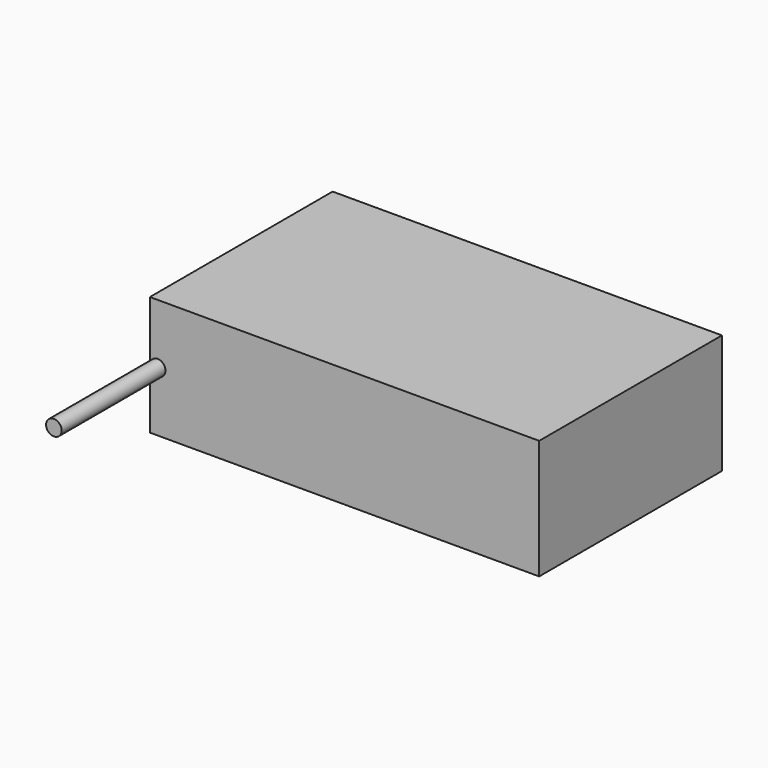
from build123d import *

# Parameters (mm, degrees)
F1_DEPTH = 23
F3_DEPTH = 25


# Not quite as in the source:
# - the program builds the solid bodies; features that only make, move or delete a surface that nothing else refers to are left out


with BuildPart() as f1:
    # F0 (on Top) → F1 (new body)
    with BuildSketch(Plane.XY):
        Polygon((-37.5, 22), (-37.5, -22), (-15.1, -22), (37.5, -22), (37.5, 22), (-15.1, 22), align=None)
    extrude(amount=F1_DEPTH)

    # F2 (on face) → F3 (join)
    with BuildSketch(Plane.XZ.offset(22)):
        with BuildLine():
            ThreePointArc((-37.5, 11.5), (-36, 10), (-34.5, 11.5))
            ThreePointArc((-34.5, 11.5), (-36, 13), (-37.5, 11.5))
        make_face()
    extrude(amount=F3_DEPTH)


solid = f1.part
